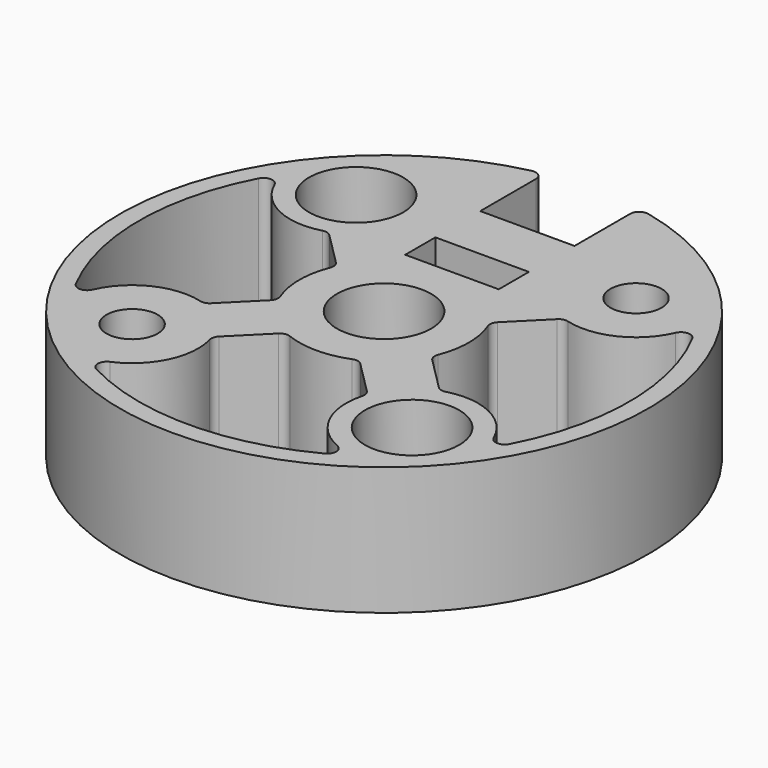
from build123d import *

# Parameters (mm, degrees)
F0_R            = 2.15265
F0_R_2          = 3.96875
F0_W            = 7.874
F0_H            = 3.175
F1_DEPTH        = 10.795
F2_R            = 1.8288
F3_REACH        = 42.4798775257
F5_R            = 3.96875
F6_DEPTH        = 4.445
F8_DEPTH        = 10.795
F8_COPIES_COUNT = 3
F8_COPIES_ANGLE = 180
F9_R            = 0.762
F11_R           = 3.96875
F11_R_2         = 2.15265
F13_DEPTH       = 6.35


# Not quite as in the source:
# - a feature of the source that left no trace in its solid (it failed there, or was rolled back) is left out
# - a pattern or mirror of a feature is missing from the dataset's text; its kind, count and spacing are read off the source's solid


with BuildPart() as f1:
    # F0 (on Top) → F1 (new body)
    with BuildSketch(Plane.XY):
        with BuildLine():
            Line((3.96875, 15.08125), (-3.96875, 15.08125))
            Line((-3.96875, 15.08125), (-3.96875, 21.8677764859))
            ThreePointArc((-3.96875, 21.8677764859), (0, -22.225), (3.96875, 21.8677764859))
            Line((3.96875, 21.8677764859), (3.96875, 15.08125))
        make_face()
        with Locations((-11.7865861589, -11.7865861589)):
            Circle(F0_R, mode=Mode.SUBTRACT)
        with Locations((11.7865861589, -11.7865861589)):
            Circle(F0_R, mode=Mode.SUBTRACT)
        with Locations((-11.7865861589, 11.7865861589)):
            Circle(F0_R, mode=Mode.SUBTRACT)
        Circle(F0_R_2, mode=Mode.SUBTRACT)
        with Locations((0, 8.73125)):
            Rectangle(F0_W, F0_H, mode=Mode.SUBTRACT)
        with Locations((11.7865861589, 11.7865861589)):
            Circle(F0_R, mode=Mode.SUBTRACT)
    extrude(amount=F1_DEPTH)

    f3_end = f1.faces().sort_by_distance((-3.96875, 0, 5.3975))[0]
    # F2 (on face) → F3 (cut, up to a face of the model that its end follows)
    with BuildSketch(Plane(origin=(0, 15.08125, 0), x_dir=(-1, 0, 0), z_dir=(0, 1, 0))):
        with Locations((0, 5.3975)):
            Circle(F2_R)
    f3_long = extrude(amount=-F3_REACH, mode=Mode.PRIVATE)
    add(split(f3_long, bisect_by=f3_end, keep=Keep.ALL, mode=Mode.PRIVATE).solids().sort_by_distance((0, 15.08125, 5.3975))[0], mode=Mode.SUBTRACT)

    # F5 (on face) → F6 (cut, through all)
    with BuildSketch(Plane(origin=(0, 0, 0), x_dir=(1, 0, 0), z_dir=(0, 0, -1))):
        with Locations((11.7865861589, -11.7865861589)):
            Circle(F5_R)
        with Locations((-11.7865861589, 11.7865861589)):
            Circle(F5_R)
    extrude(amount=-F6_DEPTH, mode=Mode.SUBTRACT)

    # F7 (on face) → F8 (cut, through all)
    with BuildSketch(Plane(origin=(0, 0, 0), x_dir=(1, 0, 0), z_dir=(0, 0, -1))):
        with BuildLine():
            ThreePointArc((-17.3148424047, -11.229543123), (-14.7565267097, -7.0906978311), (-9.9206262673, -6.5530302219))
            Line((-9.9206262673, -6.5530302219), (-6.4462980227, -3.0787019773))
            ThreePointArc((-6.4462980227, -3.0787019773), (-7.14375, 0), (-6.4462980227, 3.0787019773))
            Line((-6.4462980227, 3.0787019773), (-9.9206262673, 6.5530302219))
            ThreePointArc((-9.9206262673, 6.5530302219), (-14.7565267097, 7.0906978311), (-17.3148424047, 11.229543123))
            ThreePointArc((-17.3148424047, 11.229543123), (-20.6375, 0), (-17.3148424047, -11.229543123))
        make_face()
    f8 = extrude(amount=-F8_DEPTH, mode=Mode.SUBTRACT)

    # F8_copies: F8 ×3 about axis
    f8_copies_axis = Axis((0, 0, 0), (0, 0, 1))
    for i in range(1, F8_COPIES_COUNT):
        add(f8.rotate(f8_copies_axis, i * F8_COPIES_ANGLE / (F8_COPIES_COUNT - 1)), mode=Mode.SUBTRACT)

    # F9
    f9_edges = [f1.edges().sort_by_distance(p)[0] for p in [
        (-17.314842, -11.229543, 5.3975),
        (-9.920626, -6.55303, 5.3975),
        (-6.446298, -3.078702, 5.3975),
        (-6.446298, 3.078702, 5.3975),
        (-9.920626, 6.55303, 5.3975),
        (-17.314842, 11.229543, 5.3975),
        (3.96875, 21.867776, 5.3975),
        (-3.96875, 21.867776, 5.3975),
        (11.229543, -17.314842, 5.3975),
        (-11.229543, -17.314842, 5.3975),
        (6.55303, -9.920626, 5.3975),
        (-6.55303, -9.920626, 5.3975),
        (3.078702, -6.446298, 5.3975),
        (-3.078702, -6.446298, 5.3975),
        (17.314842, 11.229543, 5.3975),
        (17.314842, -11.229543, 5.3975),
        (9.920626, 6.55303, 5.3975),
        (6.446298, 3.078702, 5.3975),
        (6.446298, -3.078702, 5.3975),
        (9.920626, -6.55303, 5.3975),
    ]]
    fillet(f9_edges, radius=F9_R)

    # F11 (on face) → F13 (cut, through all)
    with BuildSketch(Plane.XY.offset(10.795)):
        with Locations((-11.7865861589, 11.7865861589)):
            Circle(F11_R)
        with Locations((-11.7865861589, 11.7865861589)):
            Circle(F11_R_2, mode=Mode.SUBTRACT)
        with Locations((11.7865861589, -11.7865861589)):
            Circle(F11_R)
        with Locations((11.7865861589, -11.7865861589)):
            Circle(F11_R_2, mode=Mode.SUBTRACT)
    extrude(amount=-F13_DEPTH, mode=Mode.SUBTRACT)


solid = f1.part
